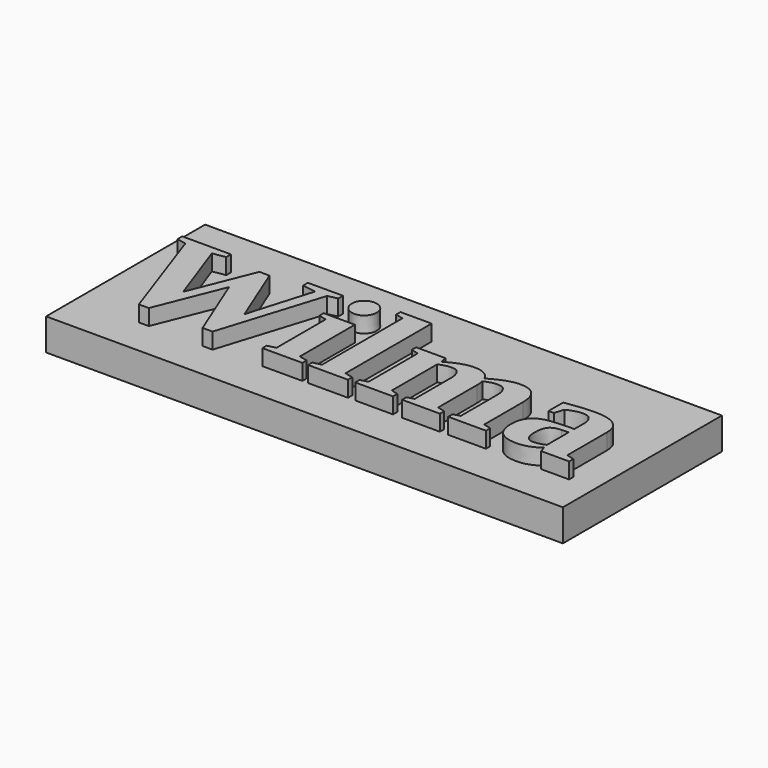
from build123d import *

# Parameters (mm, degrees)
F0_W         = 130
F0_H         = 50
F1_DEPTH     = 8
F2_TEXT_SIZE = 41.6666666667
F3_DEPTH     = 4


# Not quite as in the source:
# - Text() gives the source's letters only with a copy of the font that has no kerning and outlines rounded to 1/6400 em; it was checked with that copy


with BuildPart() as f1:
    # F0 (on Top) → F1 (new body)
    with BuildSketch(Plane.XY):
        with Locations((65, 25)):
            Rectangle(F0_W, F0_H)
    extrude(amount=F1_DEPTH)

    # F2 (on face) → F3 (join)
    with BuildSketch(Plane.XY.offset(8)):
        with Locations((3.8346354167, 10)):
            Text('Wilma', F2_TEXT_SIZE, font='Tinos', font_style=FontStyle.BOLD, text_align=(TextAlign.LEFT, TextAlign.BOTTOM))
    extrude(amount=F3_DEPTH)


solid = f1.part
